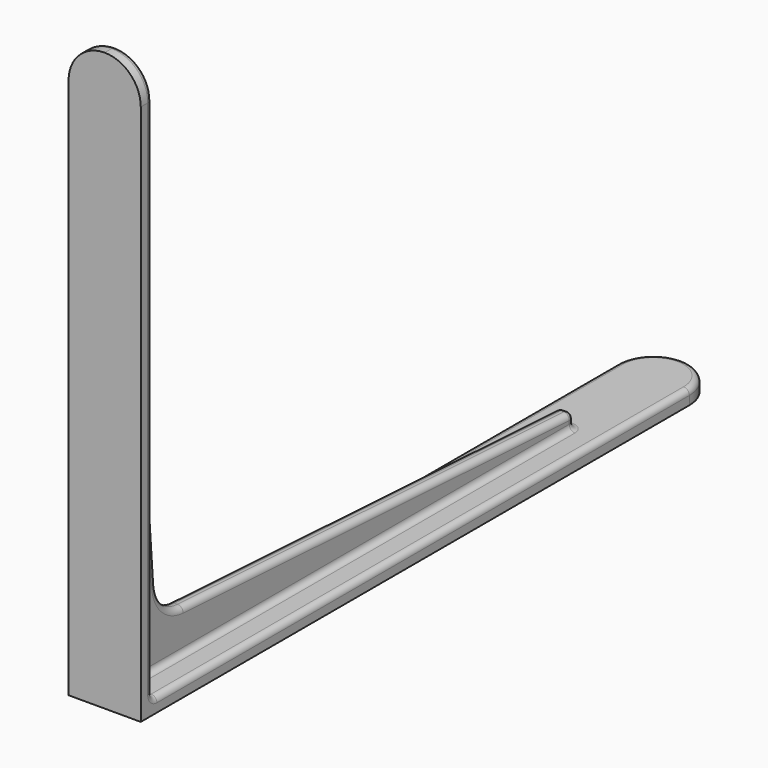
from build123d import *

# Parameters (mm, degrees)
F1_DEPTH = 25
F4_DEPTH = 5
F5_R     = 12.49999
F6_R     = 2


# Not quite as in the source:
# - a fillet or chamfer is up to 0.001 mm smaller than in the source, because OpenCascade refuses the exact size


with BuildPart() as f1:
    # F0 (on Right) → F1 (new body)
    with BuildSketch(Plane.YZ):
        Polygon((0, 200), (0, 0), (250, 0), (250, 5), (5, 5), (5, 200), align=None)
    extrude(amount=-F1_DEPTH)

    # F3 (on offset) → F4 (join)
    with BuildSketch(Plane.YZ.offset(-10)):
        Polygon((10, 150), (5, 150), (5, 5), (200, 5), (200, 10), (20, 20), align=None)
    extrude(amount=-F4_DEPTH)

    # F5 (radius 12.5 in the source; OpenCascade refuses exactly that, so slightly less here)
    f5_edges = [f1.edges().sort_by_distance(p)[0] for p in [
        (0, 2.5, 200),
        (-25, 2.5, 200),
        (-25, 250, 2.5),
        (0, 250, 2.5),
        (-12.5, 20, 20),
    ]]
    fillet(f5_edges, radius=F5_R)

    # F6
    f6_edges = [f1.edges().sort_by_distance(p)[0] for p in [
        (0, 5, 96.250005),
        (-3.661162, 5, 196.338838),
        (-5, 5, 5),
        (-12.5, 5, 200),
        (-10, 5, 77.5),
        (-21.338838, 5, 196.338838),
        (-12.5, 5, 150),
        (-25, 5, 96.250005),
        (-15, 5, 77.5),
        (-20, 5, 5),
        (-10, 14.5802, 90.457403),
        (-12.5, 19.1604, 30.914806),
        (-12.5, 10, 150),
        (-15, 14.5802, 90.457403),
        (-15, 115.465098, 14.696383),
        (-15, 22.879257, 22.94117),
        (-15, 200, 7.5),
        (-15, 102.5, 5),
        (-15, 7.5, 150),
        (-10, 115.465098, 14.696383),
        (-10, 22.879257, 22.94117),
        (-10, 200, 7.5),
        (-10, 102.5, 5),
        (-10, 7.5, 150),
        (0, 121.250005, 5),
        (-3.661162, 246.338838, 5),
        (-12.5, 250, 5),
        (-21.338838, 246.338838, 5),
        (-12.5, 200, 5),
        (-25, 121.250005, 5),
        (-12.5, 200, 10),
    ]]
    fillet(f6_edges, radius=F6_R)


solid = f1.part
